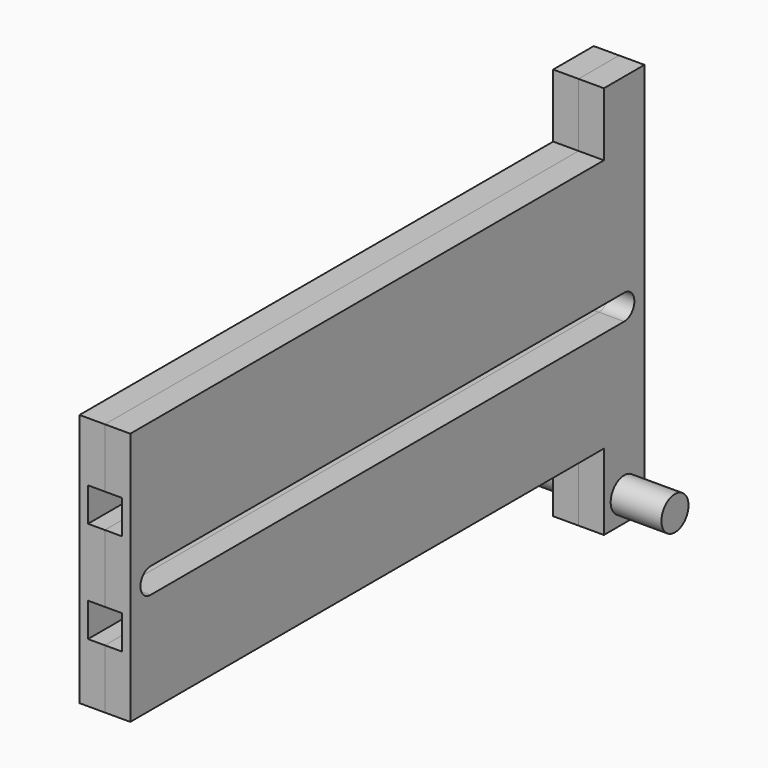
from build123d import *

# Parameters (mm, degrees)
F0_W      = 3
F0_H      = 30
F1_DEPTH  = 76
F3_W      = 2
F3_H      = 4
F7_W      = 2
F7_H      = 4
F2_R      = 2
F10_DEPTH = 2
F11_DEPTH = 3.001
F13_DEPTH = 2
F14_W     = 3
F14_H     = 6
F15_DEPTH = 7.5
F16_W     = 3
F16_H     = 6
F17_DEPTH = 9
F18_R     = 2
F19_DEPTH = 6


# Not quite as in the source:
# - a feature names something its author has since deleted; it is built from what else it names


with BuildPart() as f1:
    # F0 (on Front) → F1 (new body)
    with BuildSketch(Plane.XZ):
        Rectangle(F0_W, F0_H)
    extrude(amount=F1_DEPTH)

    # F4: sweep along a path in F2
    with BuildLine(Plane.YZ.offset(1.5)) as f4_path:
        Line((-76, -6), (-68.9066729089, -6))
        ThreePointArc((-68.9066729089, -6), (-68.0145488814, -6.0802322494), (-67.1510557009, -6.3183541122))
        Line((-67.1510557009, -6.3183541122), (-60.4069723837, -8.8473853561))
        ThreePointArc((-60.4069723837, -8.8473853561), (-59.9949330402, -8.9818373205), (-59.572797851, -9.0801004029))
        Line((-59.572797851, -9.0801004029), (-52, -10.5))
    # F3 (on face) → F4 (sweep, cut)
    with BuildSketch(Plane.XZ.offset(76)):
        with Locations((0.5, -6)):
            Rectangle(F3_W, F3_H)
    sweep(path=f4_path.line, mode=Mode.SUBTRACT)

    # F5: sweep along a path in F2
    with BuildLine(Plane.YZ.offset(1.5)) as f5_path:
        Line((-76, 6), (-68, 6))
        Line((-68, 6), (-60.4647009935, 6))
        ThreePointArc((-60.4647009935, 6), (-60.0019941065, 6.0214558015), (-59.5432583182, 6.0856390653))
        Line((-59.5432583182, 6.0856390653), (-52, 7.5))
    # F3 (on face) → F5 (sweep, cut)
    with BuildSketch(Plane.XZ.offset(76)):
        with Locations((0.5, 6)):
            Rectangle(F3_W, F3_H)
    sweep(path=f5_path.line, mode=Mode.SUBTRACT)

    # F8: sweep along a path in F2
    with BuildLine(Plane.YZ.offset(1.5)) as f8_path:
        Line((-24, -6), (-16.9066729089, -6))
        ThreePointArc((-16.9066729089, -6), (-16.0145488814, -6.0802322494), (-15.1510557009, -6.3183541122))
        Line((-15.1510557009, -6.3183541122), (-8.4069723837, -8.8473853561))
        ThreePointArc((-8.4069723837, -8.8473853561), (-7.9949330402, -8.9818373205), (-7.572797851, -9.0801004029))
        Line((-7.572797851, -9.0801004029), (0, -10.5))
    # F7 (on offset) → F8 (sweep, cut)
    with BuildSketch(Plane.XZ.offset(24)):
        with Locations((0.5, -6)):
            Rectangle(F7_W, F7_H)
    sweep(path=f8_path.line, mode=Mode.SUBTRACT)

    # F9: sweep along a path in F2
    with BuildLine(Plane.YZ.offset(1.5)) as f9_path:
        Line((-24, 6), (-16, 6))
        Line((-16, 6), (-8.4647009935, 6))
        ThreePointArc((-8.4647009935, 6), (-8.0019941065, 6.0214558015), (-7.5432583182, 6.0856390653))
        Line((-7.5432583182, 6.0856390653), (0, 7.5))
    # F7 (on offset) → F9 (sweep, cut)
    with BuildSketch(Plane.XZ.offset(24)):
        with Locations((0.5, 6)):
            Rectangle(F7_W, F7_H)
    sweep(path=f9_path.line, mode=Mode.SUBTRACT)

    # F2 (on face) → F10 (cut)
    with BuildSketch(Plane.YZ.offset(1.5)):
        with BuildLine():
            ThreePointArc((-50, 7.5), (-52.1850827548, 9.4914176794), (-53.9657443739, 7.1314229299))
            ThreePointArc((-53.9657443739, 7.1314229299), (-51.8149172452, 5.5085823206), (-50, 7.5))
        make_face()
        with BuildLine():
            ThreePointArc((-50, -10.5), (-51.8149172452, -8.5085823206), (-53.9657443739, -10.1314229299))
            ThreePointArc((-53.9657443739, -10.1314229299), (-52.1850827548, -12.4914176794), (-50, -10.5))
        make_face()
        with BuildLine():
            Line((0, 7.5), (0, 9.5))
            ThreePointArc((0, 9.5), (-1.5390182163, 8.7772716743), (-1.9657443739, 7.1314229299))
            Line((-1.9657443739, 7.1314229299), (0, 7.5))
        make_face()
        with BuildLine():
            ThreePointArc((-1.9657443739, -10.1314229299), (-1.5390182163, -11.7772716743), (0, -12.5))
            Line((0, -12.5), (0, -10.5))
            Line((0, -10.5), (-1.9657443739, -10.1314229299))
        make_face()
        with Locations((-24, 6)):
            Circle(F2_R)
        with Locations((-24, -6)):
            Circle(F2_R)
    extrude(amount=-F10_DEPTH, mode=Mode.SUBTRACT)

    # F2 (on face) → F11 (cut, through all)
    with BuildSketch(Plane.YZ.offset(1.5)):
        with BuildLine():
            Line((-38, 0), (-73, 0))
            ThreePointArc((-73, 0), (-74.5, -1.5), (-73, -3))
            Line((-73, -3), (-38, -3))
            Line((-38, -3), (-38, 0))
        make_face()
        with BuildLine():
            Line((-3, 0), (-38, 0))
            Line((-38, 0), (-38, -3))
            Line((-38, -3), (-3, -3))
            ThreePointArc((-3, -3), (-1.5, -1.5), (-3, 0))
        make_face()
    extrude(amount=-F11_DEPTH, mode=Mode.SUBTRACT)

    # F12 (on face) → F13 (cut)
    with BuildSketch(Plane(origin=(0, 0, 0), x_dir=(1, 0, 0), z_dir=(0, 0, -1))):
        Polygon((1.5, 38), (1.5, 73), (0, 73), (0, 63), (0.9, 59), (0.9, 38), align=None)
        Polygon((1.5, 3), (1.5, 38), (0.9, 38), (0, 38), (0, 28), (0.9, 24), (0.9, 3), align=None)
    extrude(amount=-F13_DEPTH, mode=Mode.SUBTRACT)

    # F14 (on face) → F15 (join)
    with BuildSketch(Plane.XY.offset(15)):
        with Locations((0, -3)):
            Rectangle(F14_W, F14_H)
    extrude(amount=F15_DEPTH)

    # F16 (on face) → F17 (join)
    with BuildSketch(Plane(origin=(0, 0, -15), x_dir=(1, 0, 0), z_dir=(0, 0, -1))):
        with Locations((0, 3)):
            Rectangle(F16_W, F16_H)
    extrude(amount=F17_DEPTH)

    # F18 (on face) → F19 (join)
    with BuildSketch(Plane(origin=(-1.5, 0, 0), x_dir=(0, -1, 0), z_dir=(-1, 0, 0))):
        with Locations((3, -21)):
            Circle(F18_R)
    extrude(amount=F19_DEPTH)


with BuildPart() as f20_1:
    # F20: instance of F1
    add(f1.part.mirror(Plane(origin=(1.5, -35.8541868499, 0.1982615546), x_dir=(0, 1, 0), z_dir=(1, 0, 0))))


solid = Compound([f1.part, f20_1.part])
